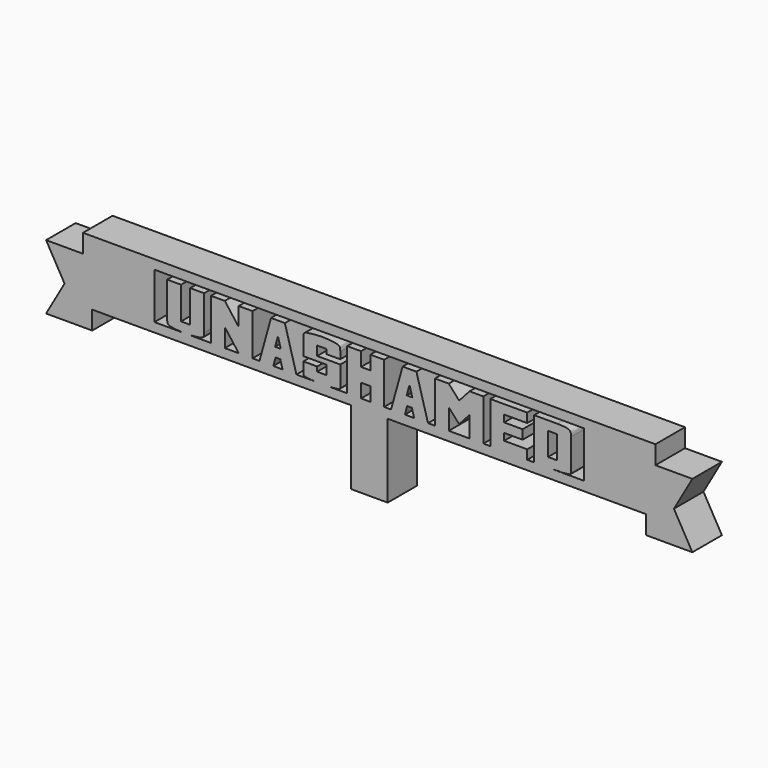
from build123d import *

# Parameters (mm, degrees)
F0_W     = 6.35
F0_H     = 9.525
F0_W_2   = 1.5875
F0_H_2   = 3.96875
F0_H_3   = 3.175
F1_DEPTH = 6.35


# Not quite as in the source:
# - a length typed as a fraction of an inch, garbled in the dataset ("3 / 203.2 mm" for 3/8 in), is restored


with BuildPart() as f1:
    # F0 (on Front) → F1 (new body)
    with BuildSketch(Plane.XZ):
        Polygon((52.4060167908, -29.36875), (55.5810167908, -23.8125), (49.2310167908, -23.8125), (49.2310167908, -20.6375), (-49.1939832092, -20.6375), (-49.1939832092, -23.8125), (-55.5439832092, -23.8125), (-52.3689832092, -29.36875), (-55.5439832092, -34.925), (-47.6064832092, -34.925), (-47.6064832092, -31.75), (-3.1564832092, -31.75), (3.1935167908, -31.75), (47.6435167908, -31.75), (47.6435167908, -34.925), (55.5810167908, -34.925), align=None)
        with BuildLine():
            Line((-36.909375, -22.225), (36.909375, -22.225))
            Line((36.909375, -22.225), (36.909375, -30.1625))
            Line((36.909375, -30.1625), (34.7265625, -30.1625))
            Line((34.7265625, -30.1625), (31.5515625, -30.1625))
            Line((31.5515625, -30.1625), (28.3765625, -30.1625))
            Line((28.3765625, -30.1625), (27.1859375, -30.1625))
            Line((27.1859375, -30.1625), (20.8359375, -30.1625))
            Line((20.8359375, -30.1625), (19.6453125, -30.1625))
            Line((19.6453125, -30.1625), (17.2640625, -30.1625))
            Line((17.2640625, -30.1625), (13.6921875, -30.1625))
            Line((13.6921875, -30.1625), (11.3109375, -30.1625))
            Line((11.3109375, -30.1625), (10.1203125, -30.1625))
            Line((10.1203125, -30.1625), (7.7390625, -30.1625))
            Line((7.7390625, -30.1625), (6.1515625, -30.1625))
            Line((6.1515625, -30.1625), (3.7703125, -30.1625))
            Line((3.7703125, -30.1625), (2.5796875, -30.1625))
            Line((2.5796875, -30.1625), (0.1984375, -30.1625))
            Line((0.1984375, -30.1625), (-1.3890625, -30.1625))
            Line((-1.3890625, -30.1625), (-3.7703125, -30.1625))
            Line((-3.7703125, -30.1625), (-4.9609375, -30.1625))
            Line((-4.9609375, -30.1625), (-6.8241157772, -30.1625))
            add(Edge.make_bspline(
                [(-8.1359375, -30.1873046875), (-7.6862010464, -30.1873046875), (-7.2364645928, -30.1795465798), (-6.8241157772, -30.1625)],
                knots=[0.5, 0.5, 0.5, 0.5, 0.5965188889, 0.5965188889, 0.5965188889, 0.5965188889], degree=3))
            add(Edge.make_bspline(
                [(-9.4477592243, -30.1625), (-9.0354104083, -30.1795465799), (-8.5856739541, -30.1873046875), (-8.1359375, -30.1873046875)],
                knots=[0.403481111, 0.403481111, 0.403481111, 0.403481111, 0.5, 0.5, 0.5, 0.5], degree=3))
            Line((-9.4477592243, -30.1625), (-11.3109375, -30.1625))
            Line((-11.3109375, -30.1625), (-12.5015625, -30.1625))
            Line((-12.5015625, -30.1625), (-14.8828125, -30.1625))
            Line((-14.8828125, -30.1625), (-16.4703125, -30.1625))
            Line((-16.4703125, -30.1625), (-18.8515625, -30.1625))
            Line((-18.8515625, -30.1625), (-20.0421875, -30.1625))
            Line((-20.0421875, -30.1625), (-22.4234375, -30.1625))
            Line((-22.4234375, -30.1625), (-24.8046875, -30.1625))
            Line((-24.8046875, -30.1625), (-27.1859375, -30.1625))
            Line((-27.1859375, -30.1625), (-28.3765625, -30.1625))
            Line((-28.3765625, -30.1625), (-30.8380988479, -30.1625))
            add(Edge.make_bspline(
                [(-31.5515625, -30.1873046875), (-31.3115619086, -30.1873046875), (-31.0715613172, -30.1779187981), (-30.8380988479, -30.1625)],
                knots=[0.5, 0.5, 0.5, 0.5, 0.5625917967, 0.5625917967, 0.5625917967, 0.5625917967], degree=3))
            add(Edge.make_bspline(
                [(-32.2650261503, -30.1625), (-32.0315636815, -30.177918798), (-31.7915630907, -30.1873046875), (-31.5515625, -30.1873046875)],
                knots=[0.4374082034, 0.4374082034, 0.4374082034, 0.4374082034, 0.5, 0.5, 0.5, 0.5], degree=3))
            Line((-32.2650261503, -30.1625), (-34.7265625, -30.1625))
            Line((-34.7265625, -30.1625), (-36.909375, -30.1625))
            Line((-36.909375, -30.1625), (-36.909375, -22.225))
        make_face(mode=Mode.SUBTRACT)
        with Locations((0.0185167908, -39.6875)):
            Rectangle(F0_W, F0_H)
        Polygon((17.2640625, -30.1625), (19.6453125, -30.1625), (19.6453125, -23.01875), (17.2640625, -23.01875), (15.478125, -25.0092855764), (13.6921875, -23.01875), (11.3109375, -23.01875), (11.3109375, -30.1625), (13.6921875, -30.1625), (13.6921875, -26.5844644236), (15.478125, -28.575), (17.2640625, -26.5844644236), align=None)
        with BuildLine():
            Line((28.3765625, -30.1625), (31.5515625, -30.1625))
            add(Edge.make_bspline(
                [(31.5515625, -30.1625), (32.7421875004, -30.1591077376), (34.5123349703, -30.1090597393), (34.7058178423, -29.8567694785), (34.7265625, -29.765625)],
                knots=[0, 0, 0, 0, 0.5486856078, 0.7169739211, 0.7169739211, 0.7169739211, 0.7169739211], degree=3))
            Line((34.7265625, -29.765625), (34.7265625, -28.971875))
            Line((34.7265625, -28.971875), (34.7265625, -24.209375))
            add(Edge.make_bspline(
                [(32.338456939, -23.01875), (33.0698998056, -23.0207151841), (33.9016308923, -23.0447678149), (34.6240389102, -23.3694667004), (34.7265625, -23.8125000002), (34.7265625, -24.209375)],
                knots=[0.1152880959, 0.1152880959, 0.1152880959, 0.1152880959, 0.4729542068, 0.722889892, 1, 1, 1, 1], degree=3))
            Line((32.338456939, -23.01875), (31.5515625, -23.01875))
            Line((31.5515625, -23.01875), (28.3765625, -23.01875))
            Line((28.3765625, -23.01875), (28.3765625, -30.1625))
        make_face()
        with Locations((31.5515625, -26.590625)):
            Rectangle(F0_W_2, F0_H_2, mode=Mode.SUBTRACT)
        Polygon((-27.1859375, -23.01875), (-27.1859375, -30.1625), (-24.8046875, -30.1625), (-24.8046875, -26.9875), (-22.4234375, -30.1625), (-20.0421875, -30.1625), (-20.0421875, -23.01875), (-22.4234375, -23.01875), (-22.4234375, -26.19375), (-24.8046875, -23.01875), align=None)
        Polygon((0.1984375, -30.1625), (2.5796875, -30.1625), (2.5796875, -23.01875), (0.1984375, -23.01875), (0.1984375, -25.4), (-1.3890625, -25.4), (-1.3890625, -23.01875), (-3.7703125, -23.01875), (-3.7703125, -30.1625), (-1.3890625, -30.1625), (-1.3890625, -27.78125), (0.1984375, -27.78125), align=None)
        with BuildLine():
            add(Edge.make_bspline(
                [(-34.7265625, -28.971875), (-34.7265625, -29.3687499998), (-34.6194398399, -29.8515743848), (-33.9447907089, -29.9651114553), (-32.920864157, -30.119185827), (-32.2650261503, -30.1625)],
                knots=[0, 0, 0, 0, 0.139450599, 0.2615766049, 0.4374082034, 0.4374082034, 0.4374082034, 0.4374082034], degree=3))
            Line((-32.2650261503, -30.1625), (-31.5515625, -30.1625))
            Line((-31.5515625, -30.1625), (-30.8380988479, -30.1625))
            add(Edge.make_bspline(
                [(-30.8380988479, -30.1625), (-30.1822608419, -30.119185827), (-29.1583342909, -29.9651114555), (-28.4836851601, -29.851574384), (-28.3765625, -29.3687500019), (-28.3765625, -28.971875)],
                knots=[0.5625917967, 0.5625917967, 0.5625917967, 0.5625917967, 0.7384233951, 0.860549401, 1, 1, 1, 1], degree=3))
            Line((-28.3765625, -28.971875), (-28.3765625, -23.01875))
            Line((-28.3765625, -23.01875), (-30.7578125, -23.01875))
            Line((-30.7578125, -23.01875), (-30.7578125, -28.575))
            Line((-30.7578125, -28.575), (-32.3453125, -28.575))
            Line((-32.3453125, -28.575), (-32.3453125, -23.01875))
            Line((-32.3453125, -23.01875), (-34.7265625, -23.01875))
            Line((-34.7265625, -23.01875), (-34.7265625, -28.971875))
        make_face()
        with BuildLine():
            add(Edge.make_bspline(
                [(-11.3109375, -29.765625), (-11.2890563147, -29.8564083098), (-11.1398834343, -30.0383555662), (-10.2076153949, -30.1310873988), (-9.4477592243, -30.1625)],
                knots=[0.1414902381, 0.1414902381, 0.1414902381, 0.1414902381, 0.2256208371, 0.403481111, 0.403481111, 0.403481111, 0.403481111], degree=3))
            Line((-9.4477592243, -30.1625), (-8.1359375, -30.1625))
            Line((-8.1359375, -30.1625), (-6.8241157772, -30.1625))
            add(Edge.make_bspline(
                [(-6.8241157772, -30.1625), (-6.0642596059, -30.1310873988), (-5.1319915657, -30.0383555662), (-4.9828186853, -29.8564083099), (-4.9609375, -29.765625)],
                knots=[0.5965188889, 0.5965188889, 0.5965188889, 0.5965188889, 0.7743791629, 0.8585097619, 0.8585097619, 0.8585097619, 0.8585097619], degree=3))
            Line((-4.9609375, -29.765625), (-4.9609375, -28.971875))
            Line((-4.9609375, -28.971875), (-4.9609375, -26.19375))
            Line((-4.9609375, -26.19375), (-8.9296875, -26.19375))
            Line((-8.9296875, -26.19375), (-8.9296875, -24.60625))
            Line((-8.9296875, -24.60625), (-7.3421875, -24.60625))
            Line((-7.3421875, -24.60625), (-7.3421875, -25.4))
            Line((-7.3421875, -25.4), (-4.9609375, -25.4))
            Line((-4.9609375, -25.4), (-4.9609375, -24.209375))
            add(Edge.make_bspline(
                [(-8.1359375, -23.01875), (-7.2216783904, -23.0187499999), (-5.8389001857, -23.1942073937), (-5.0681026979, -23.3310171279), (-4.9609375, -23.8124999986), (-4.9609375, -24.209375)],
                knots=[0.5, 0.5, 0.5, 0.5, 0.738366324, 0.8605189755, 1, 1, 1, 1], degree=3))
            add(Edge.make_bspline(
                [(-11.3109375, -24.209375), (-11.3109375, -23.8125000002), (-11.2037723021, -23.3310171272), (-10.4329748143, -23.194207394), (-9.0501966096, -23.0187500001), (-8.1359375, -23.01875)],
                knots=[0, 0, 0, 0, 0.1394810245, 0.261633676, 0.5, 0.5, 0.5, 0.5], degree=3))
            Line((-11.3109375, -24.209375), (-11.3109375, -26.9875))
            Line((-11.3109375, -26.9875), (-7.3421875, -26.9875))
            Line((-7.3421875, -26.9875), (-7.3421875, -28.575))
            Line((-7.3421875, -28.575), (-8.9296875, -28.575))
            Line((-8.9296875, -28.575), (-8.9296875, -27.78125))
            Line((-8.9296875, -27.78125), (-11.3109375, -27.78125))
            Line((-11.3109375, -27.78125), (-11.3109375, -28.971875))
            Line((-11.3109375, -28.971875), (-11.3109375, -29.765625))
        make_face()
        Polygon((20.8359375, -30.1625), (27.1859375, -30.1625), (27.1859375, -28.575), (23.2171875, -28.575), (23.2171875, -27.384375), (26.3921875, -27.384375), (26.3921875, -25.796875), (23.2171875, -25.796875), (23.2171875, -24.60625), (27.1859375, -24.60625), (27.1859375, -23.01875), (20.8359375, -23.01875), align=None)
        Polygon((-16.8671875, -23.01875), (-18.8515625, -30.1625), (-16.4703125, -30.1625), (-16.0734375, -28.73375), (-15.2796875, -28.73375), (-14.8828125, -30.1625), (-12.5015625, -30.1625), (-14.4859375, -23.01875), align=None)
        Polygon((-16.160156063, -27.14625), (-15.6765625, -25.4053131732), (-15.192968937, -27.14625), align=None, mode=Mode.SUBTRACT)
        Polygon((7.7390625, -30.1625), (10.1203125, -30.1625), (8.1359375, -23.01875), (5.7546875, -23.01875), (3.7703125, -30.1625), (6.1515625, -30.1625), (6.5484375, -28.73375), (7.3421875, -28.73375), align=None)
        Polygon((6.461718937, -27.14625), (6.9453125, -25.4053131732), (7.428906063, -27.14625), align=None, mode=Mode.SUBTRACT)
        with Locations((0.0185167908, -33.3375)):
            Rectangle(F0_W, F0_H_3)
        with BuildLine():
            Line((-8.1359375, -30.1625), (-9.4477592243, -30.1625))
            add(Edge.make_bspline(
                [(-9.4477592243, -30.1625), (-9.0354104083, -30.1795465799), (-8.5856739541, -30.1873046875), (-8.1359375, -30.1873046875)],
                knots=[0.403481111, 0.403481111, 0.403481111, 0.403481111, 0.5, 0.5, 0.5, 0.5], degree=3))
            Line((-8.1359375, -30.1873046875), (-8.1359375, -30.1625))
        make_face()
        with BuildLine():
            Line((-6.8241157772, -30.1625), (-8.1359375, -30.1625))
            Line((-8.1359375, -30.1625), (-8.1359375, -30.1873046875))
            add(Edge.make_bspline(
                [(-8.1359375, -30.1873046875), (-7.6862010464, -30.1873046875), (-7.2364645928, -30.1795465798), (-6.8241157772, -30.1625)],
                knots=[0.5, 0.5, 0.5, 0.5, 0.5965188889, 0.5965188889, 0.5965188889, 0.5965188889], degree=3))
        make_face()
        with BuildLine():
            Line((-31.5515625, -30.1625), (-32.2650261503, -30.1625))
            add(Edge.make_bspline(
                [(-32.2650261503, -30.1625), (-32.0315636815, -30.177918798), (-31.7915630907, -30.1873046875), (-31.5515625, -30.1873046875)],
                knots=[0.4374082034, 0.4374082034, 0.4374082034, 0.4374082034, 0.5, 0.5, 0.5, 0.5], degree=3))
            Line((-31.5515625, -30.1873046875), (-31.5515625, -30.1625))
        make_face()
        with BuildLine():
            Line((-30.8380988479, -30.1625), (-31.5515625, -30.1625))
            Line((-31.5515625, -30.1625), (-31.5515625, -30.1873046875))
            add(Edge.make_bspline(
                [(-31.5515625, -30.1873046875), (-31.3115619086, -30.1873046875), (-31.0715613172, -30.1779187981), (-30.8380988479, -30.1625)],
                knots=[0.5, 0.5, 0.5, 0.5, 0.5625917967, 0.5625917967, 0.5625917967, 0.5625917967], degree=3))
        make_face()
    extrude(amount=F1_DEPTH)


solid = f1.part
